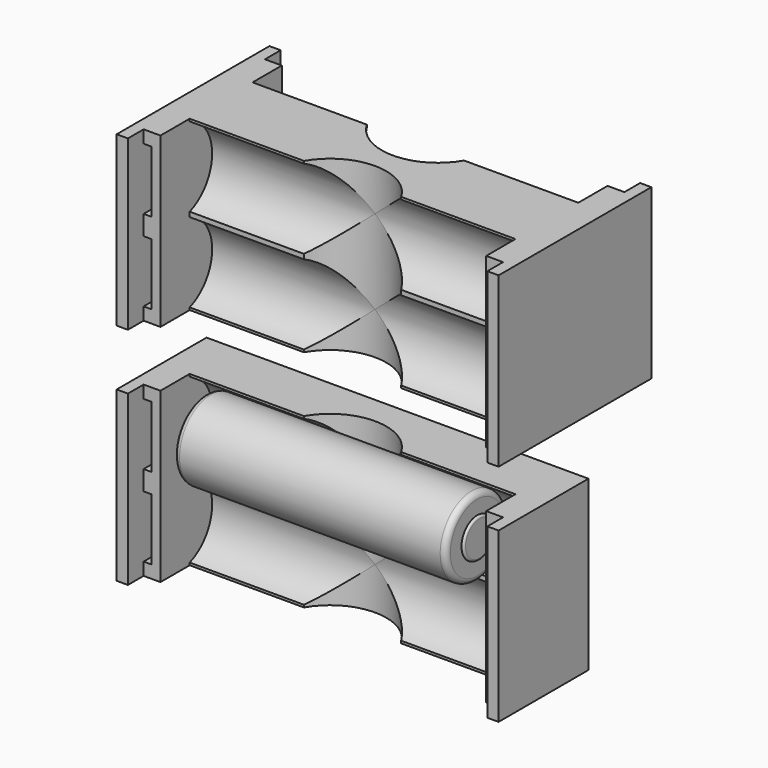
from build123d import *

# Parameters (mm, degrees)
F1_DEPTH  = 15
F2_W      = 1.4
F2_H      = 11
F3_DEPTH  = 11.5
F4_W      = 10
F4_H      = 6
F6_DEPTH  = 3
F5_W      = 1
F5_H      = 6
F7_DEPTH  = 20.001
F9_DEPTH  = 29
F13_R     = 1
F14_R     = 0.39999
F17_DEPTH = 3


# Not quite as in the source:
# - a fillet or chamfer is up to 0.001 mm smaller than in the source, because OpenCascade refuses the exact size


with BuildPart() as f1:
    # F0 (on Top) → F1 (new body, symmetric)
    with BuildSketch(Plane.XY):
        with BuildLine():
            Line((34, 10), (-34, 10))
            Line((-34, 10), (-34, -10))
            Line((-34, -10), (-32, -10))
            Line((-32, -10), (-32, -6.5))
            Line((-32, -6.5), (-29, -6.5))
            Line((-29, -6.5), (-29, 0))
            Line((-29, 0), (-8.6602540378, 0))
            ThreePointArc((-8.6602540378, 0), (0, 5), (8.6602540378, 0))
            Line((8.6602540378, 0), (29, 0))
            Line((29, 0), (29, -6.5))
            Line((29, -6.5), (32, -6.5))
            Line((32, -6.5), (32, -10))
            Line((32, -10), (34, -10))
            Line((34, -10), (34, 10))
        make_face()
    extrude(amount=F1_DEPTH, both=True)

    # F2 (on face) → F3 (cut)
    with BuildSketch(Plane.XZ.offset(6.5)):
        with Locations((-31.3, 7.25)):
            Rectangle(F2_W, F2_H)
        with Locations((-31.3, -7.25)):
            Rectangle(F2_W, F2_H)
        with Locations((31.3, -7.25)):
            Rectangle(F2_W, F2_H)
        with Locations((31.3, 7.25)):
            Rectangle(F2_W, F2_H)
    extrude(amount=-F3_DEPTH, mode=Mode.SUBTRACT)

    # F4 (on face) → F6 (cut)
    with BuildSketch(Plane(origin=(0, 10, 0), x_dir=(-1, 0, 0), z_dir=(0, 1, 0))):
        with Locations((-27, 7.25)):
            Rectangle(F4_W, F4_H)
        with Locations((-27, -7.25)):
            Rectangle(F4_W, F4_H)
        with Locations((27, -7.25)):
            Rectangle(F4_W, F4_H)
        with Locations((27, 7.25)):
            Rectangle(F4_W, F4_H)
    extrude(amount=-F6_DEPTH, mode=Mode.SUBTRACT)

    # F5 (on face) → F7 (cut, through all)
    with BuildSketch(Plane(origin=(0, 10, 0), x_dir=(-1, 0, 0), z_dir=(0, 1, 0))):
        with Locations((-31.5, 7.25)):
            Rectangle(F5_W, F5_H)
        with Locations((-31.5, -7.25)):
            Rectangle(F5_W, F5_H)
        with Locations((31.5, 7.25)):
            Rectangle(F5_W, F5_H)
        with Locations((31.5, -7.25)):
            Rectangle(F5_W, F5_H)
    extrude(amount=-F7_DEPTH, mode=Mode.SUBTRACT)

    # F8 (on Right) → F9 (cut, symmetric)
    with BuildSketch(Plane.YZ):
        with BuildLine():
            ThreePointArc((-2.5, 0), (2.8033008589, 2.1966991411), (5, 7.5))
            ThreePointArc((5, 7.5), (-7.8033008589, 12.8033008589), (-2.5, 0))
        make_face()
        with BuildLine():
            ThreePointArc((5, -7.5), (2.8033008589, -2.1966991411), (-2.5, 0))
            ThreePointArc((-2.5, 0), (-7.8033008589, -12.8033008589), (5, -7.5))
        make_face()
    extrude(amount=F9_DEPTH, both=True, mode=Mode.SUBTRACT)


with BuildPart() as f12:
    # F11 (on offset) → F12 (revolve)
    with BuildSketch(Plane.XZ.offset(3)):
        Polygon((25, 8), (-25, 8), (-25, 5.25), (-23.8, 5.25), (-23.8, 1), (24.6, 1), (24.6, 4.5), (25, 4.5), align=None)
    revolve(axis=Axis((26.4570329338, -3, 8), (1, 0, 0)))

    # F13
    f13_edges = [f12.edges().sort_by_distance(p)[0] for p in [
        (24.6, -3, 15),
        (-23.8, -3, 15),
    ]]
    fillet(f13_edges, radius=F13_R)

    # F14 (radius 0.4 in the source; OpenCascade refuses exactly that, so slightly less here)
    f14_edges = [f12.edges().sort_by_distance(p)[0] for p in [
        (25, -3, 11.5),
        (-25, -3, 10.75),
        (-23.8, -3, 14),
        (-23.8, -3, 10.75),
    ]]
    fillet(f14_edges, radius=F14_R)


with BuildPart() as f16_1:
    # F16: copy of F1
    add(f1.part.moved(Location((0, 0, 40))))

    # F17 (cut, through all): a face of the model
    f17_faces = [f16_1.faces().sort_by_distance(p)[0] for p in [
        (0, 10, 40),
    ]]
    extrude(f17_faces, amount=-F17_DEPTH, mode=Mode.SUBTRACT)

    # F18: F16_1 across plane


with BuildPart() as f16_1_1:
    add(f16_1.part)
    add(f16_1.part.mirror(Plane.XZ.offset(-7)))


solid = Compound([f1.part, f12.part, f16_1_1.part])
